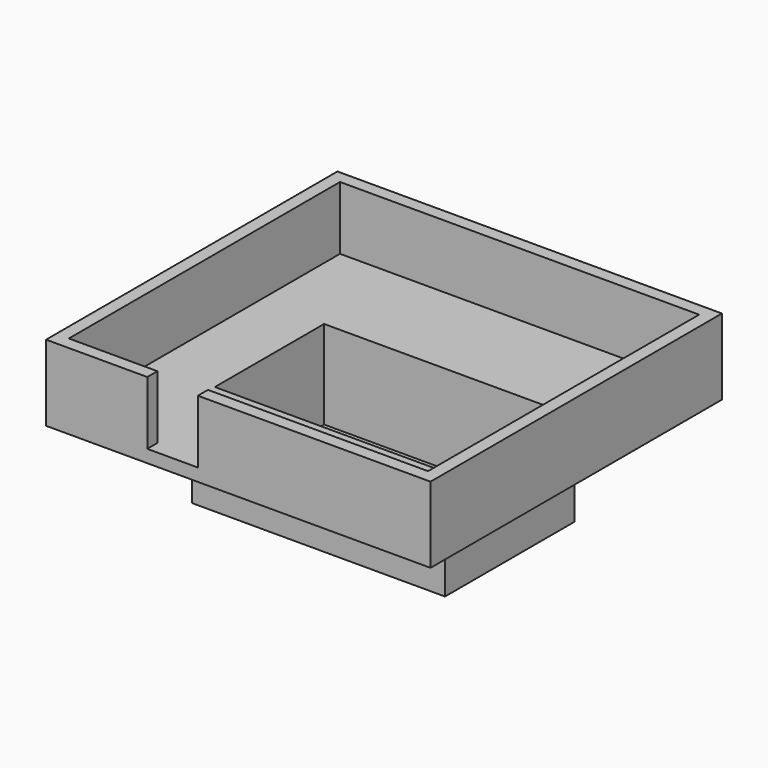
from build123d import *

# Parameters (mm, degrees)
F0_W     = 63.5
F0_H     = 40.64
F0_W_2   = 57.15
F0_H_2   = 34.29
F1_DEPTH = 3.175
F2_DEPTH = 19.05
F3_W     = 57.15
F3_H     = 34.29
F4_DEPTH = 3.175
F5_DEPTH = 19.05


# Not quite as in the source:
# - a length typed as a fraction of an inch, garbled in the dataset ("3 / 203.2 mm" for 3/8 in), is restored


with BuildPart() as f1:
    # F0 (on Top) → F1 (new body)
    with BuildSketch(Plane.XY):
        with Locations((73.5778744221, 64.3721897411)):
            Rectangle(F0_W, F0_H)
        with Locations((73.5778744221, 64.3721897411)):
            Rectangle(F0_W_2, F0_H_2, mode=Mode.SUBTRACT)
        with Locations((73.5778744221, 64.3721897411)):
            Rectangle(F0_W_2, F0_H_2)
    extrude(amount=-F1_DEPTH)

    # F0 (on Top) → F2 (join)
    with BuildSketch(Plane.XY):
        with Locations((73.5778744221, 64.3721897411)):
            Rectangle(F0_W, F0_H)
        with Locations((73.5778744221, 64.3721897411)):
            Rectangle(F0_W_2, F0_H_2, mode=Mode.SUBTRACT)
    extrude(amount=F2_DEPTH)

    # F3 (on face) → F4 (join)
    with BuildSketch(Plane.XY.offset(19.05)):
        Polygon((25.6539992988, 109.8956785083), (25.6539992988, 18.4556785083), (51.0539992988, 18.4556785083), (51.0539992988, 21.6306785083), (28.8289992988, 21.6306785083), (28.8289992988, 106.7206785083), (118.9989992988, 106.7206785083), (118.9989992988, 21.6306785083), (63.7539992988, 21.6306785083), (63.7539992988, 18.4556785083), (122.1739992988, 18.4556785083), (122.1739992988, 109.8956785083), align=None)
        Polygon((51.0539992988, 21.6306785083), (51.0539992988, 18.4556785083), (63.7539992988, 18.4556785083), (63.7539992988, 21.6306785083), (118.9989992988, 21.6306785083), (118.9989992988, 106.7206785083), (28.8289992988, 106.7206785083), (28.8289992988, 21.6306785083), align=None)
        with Locations((73.5778744221, 64.3721897411)):
            Rectangle(F3_W, F3_H, mode=Mode.SUBTRACT)
    extrude(amount=F4_DEPTH)

    # F3 (on face) → F5 (join)
    with BuildSketch(Plane.XY.offset(19.05)):
        Polygon((25.6539992988, 109.8956785083), (25.6539992988, 18.4556785083), (51.0539992988, 18.4556785083), (51.0539992988, 21.6306785083), (28.8289992988, 21.6306785083), (28.8289992988, 106.7206785083), (118.9989992988, 106.7206785083), (118.9989992988, 21.6306785083), (63.7539992988, 21.6306785083), (63.7539992988, 18.4556785083), (122.1739992988, 18.4556785083), (122.1739992988, 109.8956785083), align=None)
    extrude(amount=F5_DEPTH)


solid = f1.part
